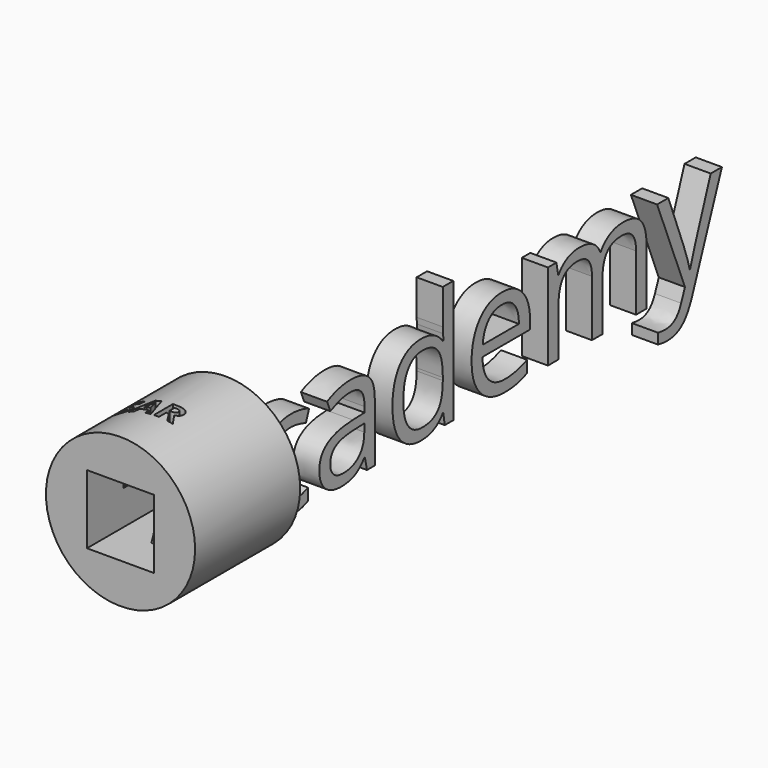
from build123d import *

# Parameters (mm, degrees)
F0_R          = 72.3811666727
F0_W          = 65.1415884495
F0_H          = 66.8011903763
F1_DEPTH      = 76.1998444796
F1_DEPTH_BACK = 51.2480810285
F2_TEXT_SIZE  = 32.2710929645
F3_DEPTH      = 150.020301342
F4_TEXT_SIZE  = 156.6759362403
F5_DEPTH      = 25.4


# Not quite as in the source:
# - Text() gives the source's letters only with a copy of the font that has no kerning and outlines rounded to 1/6400 em; it was checked with that copy


with BuildPart() as f1:
    # F0 (on Front) → F1 (new body, two sides)
    with BuildSketch(Plane.XZ) as f1_sk:
        Circle(F0_R)
        Rectangle(F0_W, F0_H, mode=Mode.SUBTRACT)
    extrude(amount=F1_DEPTH)
    extrude(f1_sk.sketch, amount=-F1_DEPTH_BACK)

    # F2 (on Top) → F3 (cut)
    with BuildSketch(Plane.XY):
        with Locations((-45.6405729055, -32.3632955551)):
            Text('SAR', F2_TEXT_SIZE, font='Open Sans', font_style=FontStyle.BOLD, text_align=(TextAlign.LEFT, TextAlign.BOTTOM))
    extrude(amount=F3_DEPTH, mode=Mode.SUBTRACT)

    # F4 (on Right) → F5 (join)
    with BuildSketch(Plane.YZ):
        with Locations((-47.7095395327, -56.3578419387)):
            Text('Academy', F4_TEXT_SIZE, font='Open Sans', text_align=(TextAlign.LEFT, TextAlign.BOTTOM))
    extrude(amount=F5_DEPTH)


solid = f1.part
